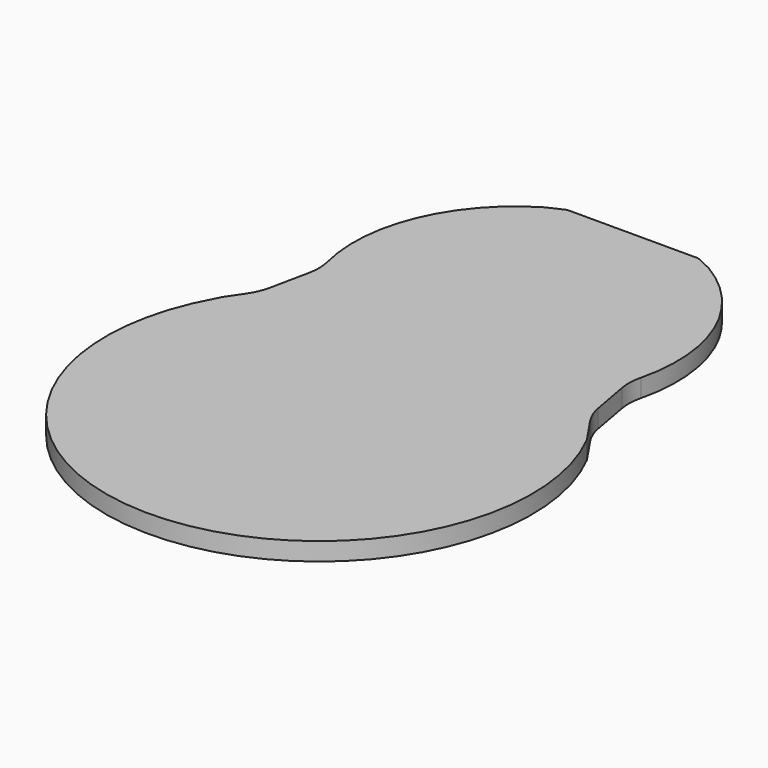
from build123d import *

# Parameters (mm, degrees)
F1_DEPTH = 6.35
F2_R     = 12.7
F4_DEPTH = 6.351


# Not quite as in the source:
# - a feature names something its author has since deleted; it is built from what else it names


with BuildPart() as f1:
    # F0 (on Top) → F1 (new body)
    with BuildSketch(Plane.XY):
        with BuildLine():
            ThreePointArc((-70.543128599, 41.1726645916), (-70.7849997477, 40.4855010306), (-71.1039826136, 39.8305618399))
            ThreePointArc((-71.1039826136, 39.8305618399), (-1.0804242799, -81.4928382336), (72.1349447987, 37.9315137965))
            Line((72.1349447987, 37.9315137965), (64.1774671745, 49.691417374))
            Line((64.1774671745, 49.691417374), (60.7204563849, 68.6290463558))
            ThreePointArc((60.7204563849, 68.6290463558), (58.8124253174, 109.8022050591), (31.9532798351, 141.0664959374))
            Line((31.9532798352, 141.0664959374), (24.5, 144.5356458426))
            Line((24.5, 144.5356458426), (0, 144.5356458426))
            Line((0, 144.5356458426), (-24.5, 144.5356458426))
            Line((-24.5, 144.5356458426), (-31.9532798352, 141.0664959374))
            ThreePointArc((-31.9532798351, 141.0664959374), (-58.8010464391, 109.8308374249), (-60.7377773112, 68.688183064))
            Line((-60.7377773112, 68.688183064), (-64.7292534015, 49.691417374))
            Line((-64.7292534015, 49.691417374), (-70.543128599, 41.1726645916))
        make_face()
    extrude(amount=F1_DEPTH)

    # F2
    f2_edges = [f1.edges().sort_by_distance(p)[0] for p in [
        (60.720456, 68.629046, 3.175),
        (72.134945, 37.931514, 3.175),
        (64.177467, 49.691417, 3.175),
        (-64.729253, 49.691417, 3.175),
        (-60.737777, 68.688183, 3.175),
    ]]
    fillet(f2_edges, radius=F2_R)

    # F3 (on face) → F4 (cut, through all)
    with BuildSketch(Plane.XY.offset(6.35)):
        with BuildLine():
            ThreePointArc((-70.543128599, 41.1726645916), (-70.7849997477, 40.4855010306), (-71.1039826136, 39.8305618399))
            ThreePointArc((-71.1039826136, 39.8305618399), (-1.4798729053, -81.4865631634), (72.5033392644, 37.2225173183))
            ThreePointArc((72.5033392644, 37.2225173183), (72.133296657, 37.8927702646), (71.7235387193, 38.5395074414))
            Line((71.7235387193, 38.5395074414), (65.673391241, 47.4806762809))
            ThreePointArc((65.673391241, 47.4806762809), (64.4343566454, 49.7963304465), (63.6981152819, 52.3173242185))
            Line((63.6981152819, 52.3173242185), (61.235654247, 65.8067740057))
            ThreePointArc((61.235654247, 65.8067740057), (61.0355921512, 68.4904493527), (61.4054899639, 71.1560288055))
            ThreePointArc((61.4054899639, 71.1560288055), (58.3166642414, 111.0138701005), (31.9532798351, 141.0664959374))
            Line((31.9532798352, 141.0664959374), (24.5, 144.5356458426))
            Line((24.5, 144.5356458426), (-24.5, 144.5356458426))
            Line((-24.5, 144.5356458426), (-31.9532798352, 141.0664959374))
            ThreePointArc((-31.9532798351, 141.0664959374), (-58.2757571875, 111.1107457801), (-61.4559677961, 71.3601980865))
            ThreePointArc((-61.4559677961, 71.3601980865), (-61.0915979292, 68.5460068659), (-61.3611887293, 65.7211602459))
            Line((-61.3611887293, 65.7211602459), (-64.2110715476, 52.1576176071))
            ThreePointArc((-64.2110715476, 52.1576176071), (-64.9570302406, 49.7885224974), (-66.149830538, 47.6099235298))
            Line((-66.149830538, 47.6099235298), (-70.543128599, 41.1726645916))
        make_face()
        with BuildLine():
            Line((-28.9966635349, 135.438502816), (-23.0945782645, 138.1856448808))
            Line((-23.0945782645, 138.1856448808), (23.0945782645, 138.1856448808))
            Line((23.0945782645, 138.1856448808), (28.9966635349, 135.438502816))
            ThreePointArc((28.9966635349, 135.438502816), (52.520857183, 108.4149325541), (55.243636, 72.6903260202))
            ThreePointArc((55.243636, 72.6903260202), (54.6887892531, 68.6919566393), (54.988882412, 64.6664434155))
            Line((54.988882412, 64.6664434155), (57.4513434469, 51.1769936283))
            ThreePointArc((57.4513434469, 51.1769936283), (58.5557055478, 47.3955027794), (60.4142575351, 43.9220213556))
            Line((60.4142575351, 43.9220213556), (66.4644050134, 34.9808525161))
            ThreePointArc((66.4644050134, 34.9808525161), (66.6692839512, 34.6574839767), (66.8543052269, 34.3223575543))
            ThreePointArc((66.8543052269, 34.3223575543), (-1.3645699068, -75.137609121), (-65.5639782212, 36.7271985762))
            ThreePointArc((-65.5639782212, 36.7271985762), (-65.1678300151, 37.4944518277), (-64.8247337429, 38.2868506548))
            Line((-64.8247337429, 38.2868506548), (-60.904901379, 44.0303662485))
            ThreePointArc((-60.904901379, 44.0303662485), (-59.1157008425, 47.2982648647), (-57.9967627465, 50.8519077088))
            Line((-57.9967627465, 50.8519077088), (-55.1468799282, 64.4154503476))
            ThreePointArc((-55.1468799282, 64.4154503476), (-54.7424937077, 68.6527204915), (-55.2890485355, 72.8740075355))
            ThreePointArc((-55.2890485355, 72.8740075355), (-52.4842770002, 108.5021804525), (-28.9966635349, 135.438502816))
        make_face(mode=Mode.SUBTRACT)
    extrude(amount=-F4_DEPTH, mode=Mode.SUBTRACT)


solid = f1.part
